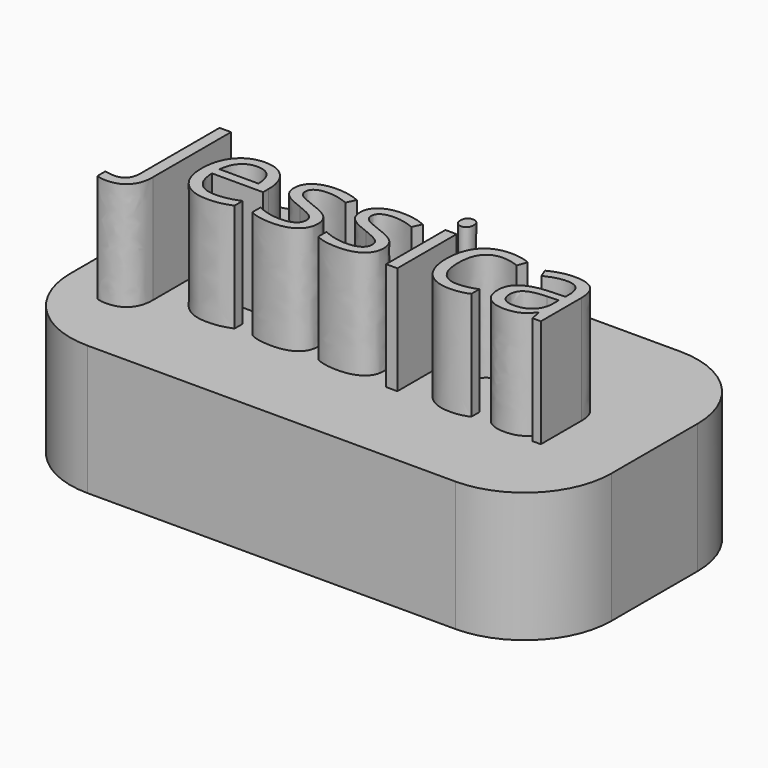
from build123d import *

# Parameters (mm, degrees)
F0_W         = 125
F0_H         = 65
F1_DEPTH     = 30
F2_TEXT_SIZE = 31.9552626323
F3_DEPTH     = 25
F5_DEPTH     = 51.3
F6_R         = 20.0379725677


# Not quite as in the source:
# - Text() gives the source's letters only with a copy of the font that has no kerning and outlines rounded to 1/6400 em; it was checked with that copy


with BuildPart() as f1:
    # F0 (on Top) → F1 (new body)
    with BuildSketch(Plane.XY):
        Rectangle(F0_W, F0_H)
    extrude(amount=F1_DEPTH)

    # F2 (on face) → F3 (join)
    with BuildSketch(Plane.XY.offset(30)):
        with Locations((-50, -11.5038945476)):
            Text('Jessica', F2_TEXT_SIZE, font='Open Sans', text_align=(TextAlign.LEFT, TextAlign.BOTTOM))
    extrude(amount=F3_DEPTH)

    # F4 (on face) → F5 (cut)
    with BuildSketch(Plane.XY.offset(30)):
        with BuildLine():
            ThreePointArc((5, 22.5), (3.5355339059, 26.0355339059), (0, 27.5))
            ThreePointArc((0, 27.5), (-3.5355339059, 18.9644660941), (5, 22.5))
        make_face()
    extrude(amount=-F5_DEPTH, mode=Mode.SUBTRACT)

    # F6
    f6_edges = [f1.edges().sort_by_distance(p)[0] for p in [
        (62.5, 32.5, 15),
        (62.5, -32.5, 15),
        (-62.5, 32.5, 15),
        (-62.5, -32.5, 15),
    ]]
    fillet(f6_edges, radius=F6_R)


solid = f1.part
